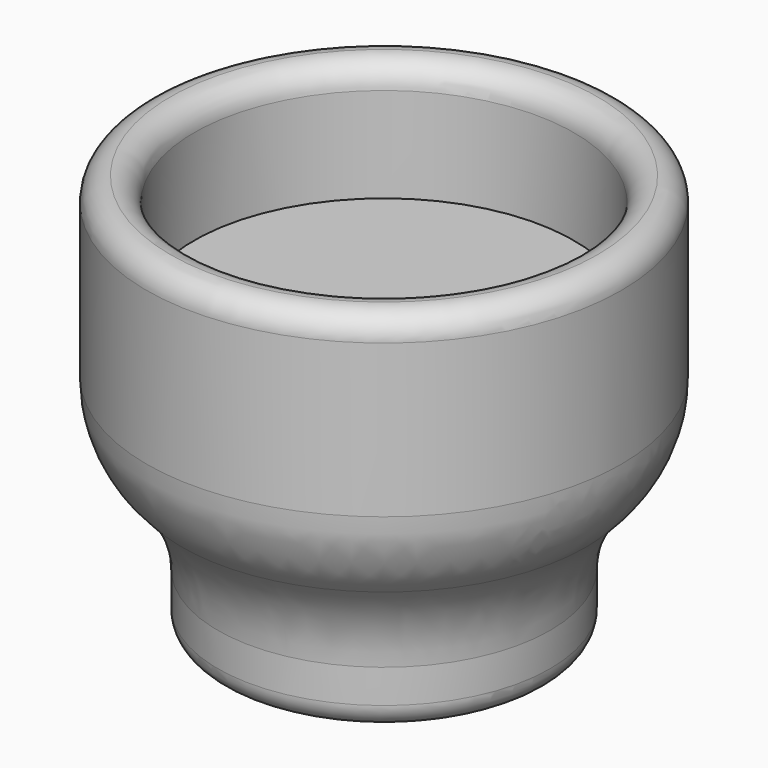
from build123d import *

# Parameters (mm, degrees)
F3_DEPTH = 7.62
F5_R     = 5
F6_R     = 0.99999
F7_R     = 0.5


# Not quite as in the source:
# - a fillet or chamfer that OpenCascade refuses, or shapes differently, is made with other operations: its cross-section is extruded or revolved along the edge and cut away or added
# - a fillet or chamfer is up to 0.001 mm smaller than in the source, because OpenCascade refuses the exact size


with BuildPart() as f1:
    # F0 (on Front) → F1 (revolve)
    with BuildSketch(Plane.XZ):
        Polygon((8, 5), (8, 0), (0, 0), (0, -12), (7, -12), (7, -5), (10, -5), (10, 5), align=None)
    revolve(axis=Axis((0, 0, -6), (0, 0, 1)))

    # F2 (on face) → F3 (cut)
    with BuildSketch(Plane(origin=(0, 0, -12), x_dir=(1, 0, 0), z_dir=(0, 0, -1))):
        Polygon((1.1547005384, 2), (-1.1547005384, 2), (-2.3094010768, 0), (-1.1547005384, -2), (1.1547005384, -2), (2.3094010768, 0), align=None)
    extrude(amount=-F3_DEPTH, mode=Mode.SUBTRACT)

    # F4: fillet of radius 5 on 1 edges, made by hand

    # F4_s1 → F4_t2 (revolve)
    with BuildSketch(Plane.XZ):
        with BuildLine():
            ThreePointArc((10, -5), (7.8166998673, -6.8439629074), (7, -9.582575695))
            Line((7, -9.582575695), (7, -5))
            Line((7, -5), (10, -5))
        make_face()
    revolve(axis=Axis((0, 0, -5), (0, 0, 1)))

    # F5
    f5_edges = [f1.edges().sort_by_distance(p)[0] for p in [
        (-10, 0, -5),
    ]]
    fillet(f5_edges, radius=F5_R)

    # F6 (radius 1 in the source; OpenCascade refuses exactly that, so slightly less here)
    f6_edges = [f1.edges().sort_by_distance(p)[0] for p in [
        (-10, 0, 5),
        (-8, 0, 5),
        (-7, 0, -12),
    ]]
    fillet(f6_edges, radius=F6_R)

    # F7
    f7_edges = [f1.edges().sort_by_distance(p)[0] for p in [
        (-2.309401, 0, -8.19),
        (-1.154701, -2, -8.19),
        (1.154701, -2, -8.19),
        (2.309401, 0, -8.19),
        (1.154701, 2, -8.19),
        (-1.154701, 2, -8.19),
    ]]
    fillet(f7_edges, radius=F7_R)


solid = f1.part
